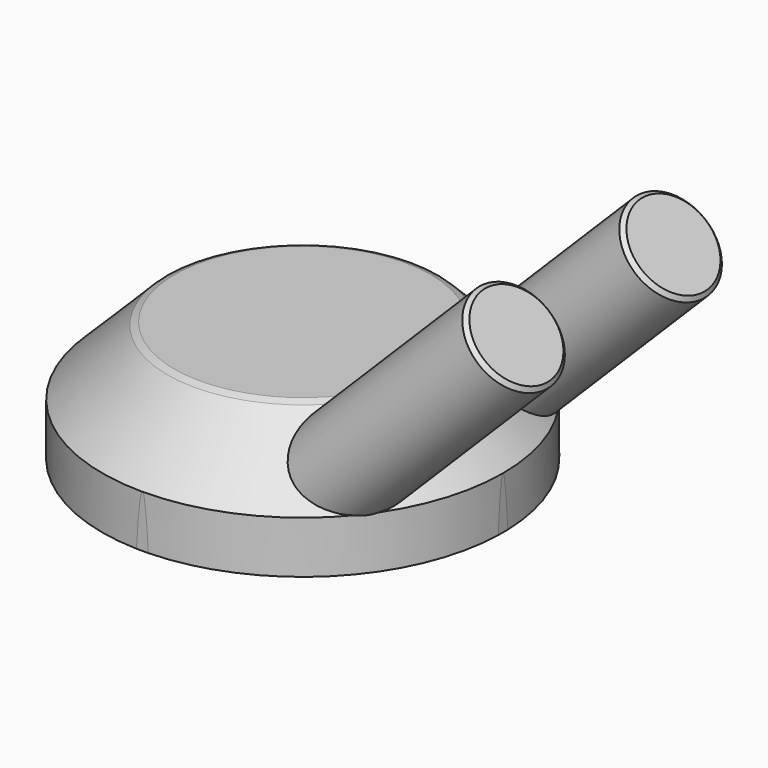
from build123d import *

# Parameters (mm, degrees)
F0_W          = 50
F0_H          = 50
F1_DEPTH      = 15
F2_SIZE       = 8.5
F3_R          = 6
F6_DEPTH      = 25
F6_DEPTH_BACK = 10
F7_SIZE       = 0.5
F7_2_SIZE     = 0.5
F7_3_SIZE     = 0.5


# Not quite as in the source:
# - a feature names something its author has since deleted; it is built from what else it names


with BuildPart() as f1:
    # F0 (on Top) → F1 (new body)
    with BuildSketch(Plane.XY):
        Rectangle(F0_W, F0_H)
    extrude(amount=-F1_DEPTH)

    # F2
    f2_edges = [f1.edges().sort_by_distance(p)[0] for p in [
        (25, 0, 0),
    ]]
    chamfer(f2_edges, length=F2_SIZE)

    # F4 (on Front) → F5 (revolve, cut)
    with BuildSketch(Plane.XZ):
        Polygon((16.5, 0), (25, -8.5), (25.0111613423, -15), (57.6415769756, -15), (57.6415769756, 0), align=None)
    revolve(axis=Axis((0, 0, -4.25), (0, 0, -1)), mode=Mode.SUBTRACT)

    # F7#3
    f7_3_edges = [f1.edges().sort_by_distance(p)[0] for p in [
        (-16.5, 0, 0),
    ]]
    chamfer(f7_3_edges, length=F7_3_SIZE)


with BuildPart() as f6:
    # F3 (on face) → F6 (new body, two sides)
    with BuildSketch(Plane(origin=(8.25, 0, 8.25), x_dir=(0, 1, 0), z_dir=(0.7071067812, 0, 0.7071067812))) as f6_sk:
        with Locations((-12.25, -14.9172618896)):
            Circle(F3_R)
    extrude(amount=F6_DEPTH)
    extrude(f6_sk.sketch, amount=-F6_DEPTH_BACK)

    # F7
    f7_edges = [f6.edges().sort_by_distance(p)[0] for p in [
        (36.475767, -18.25, 15.379572),
    ]]
    chamfer(f7_edges, length=F7_SIZE)


with BuildPart() as f6b:
    # F3 (on face) → F6, piece 2 (new body, two sides)
    with BuildSketch(Plane(origin=(8.25, 0, 8.25), x_dir=(0, 1, 0), z_dir=(0.7071067812, 0, 0.7071067812))) as f6_2_sk:
        with Locations((12.25, -14.9172618896)):
            Circle(F3_R)
    extrude(amount=F6_DEPTH)
    extrude(f6_2_sk.sketch, amount=-F6_DEPTH_BACK)

    # F7#2
    f7_2_edges = [f6b.edges().sort_by_distance(p)[0] for p in [
        (36.475767, 6.25, 15.379572),
    ]]
    chamfer(f7_2_edges, length=F7_2_SIZE)


solid = Compound([f1.part, f6.part, f6b.part])
